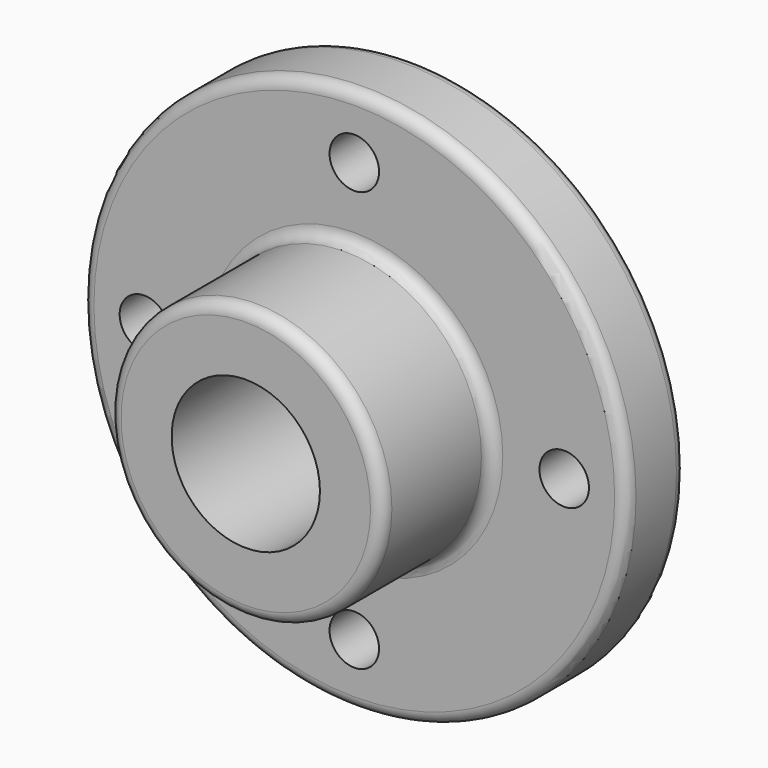
from build123d import *

# Parameters (mm, degrees)
F0_R            = 35.052
F0_R_2          = 19.0246
F1_DEPTH        = 53.848
F0_R_3          = 69.85
F0_R_4          = 53.848
F2_DEPTH        = 19.05
F3_R            = 3.048
F4_R            = 6.35
F5_DEPTH        = 19.051
F5_COPIES_COUNT = 4


# Not quite as in the source:
# - a pattern or mirror of a feature is missing from the dataset's text; its kind, count and spacing are read off the source's solid
# - a feature names something its author has since deleted; it is built from what else it names


with BuildPart() as f1:
    # F0 (on Front) → F1 (new body)
    with BuildSketch(Plane.XZ):
        Circle(F0_R)
        Circle(F0_R_2, mode=Mode.SUBTRACT)
    extrude(amount=F1_DEPTH)

    # F0 (on Front) → F2 (join)
    with BuildSketch(Plane.XZ):
        Circle(F0_R_3)
        Circle(F0_R_4, mode=Mode.SUBTRACT)
        Circle(F0_R_4)
        Circle(F0_R, mode=Mode.SUBTRACT)
    extrude(amount=F2_DEPTH)

    # F3
    f3_edges = [f1.edges().sort_by_distance(p)[0] for p in [
        (-69.85, -19.05, 0),
        (-69.85, 0, 0),
        (-35.052, -19.05, 0),
        (-35.052, -53.848, 0),
    ]]
    fillet(f3_edges, radius=F3_R)

    # F4 (on face) → F5 (cut, through all)
    with BuildSketch(Plane.XZ.offset(19.05)):
        with Locations((0, 53.848)):
            Circle(F4_R)
    f5 = extrude(amount=-F5_DEPTH, mode=Mode.SUBTRACT)

    # F5_copies: F5 ×4 about axis
    f5_copies_axis = Axis((0, 0, 0), (0, 1, 0))
    for i in range(1, F5_COPIES_COUNT):
        add(f5.rotate(f5_copies_axis, i * 360 / F5_COPIES_COUNT), mode=Mode.SUBTRACT)


solid = f1.part
